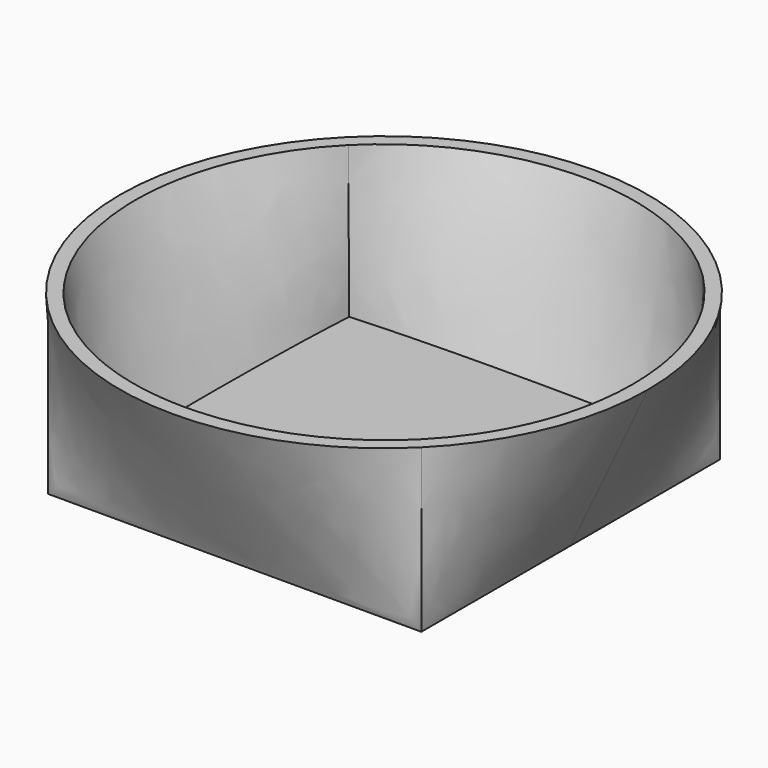
from build123d import *

# Parameters (mm, degrees)
F0_R = 48.75
F2_W = 68.9429111657
F2_H = 68.9429111657
F4_T = 2.5


# Not quite as in the source:
# - a shell that OpenCascade refuses in one call is made with other operations: the cavity is built on its own and cut out


with BuildPart() as f3:
    # F0 (on Top) → F3 section 0
    with BuildSketch(Plane.XY):
        Circle(F0_R)
    # F2 (on offset) → F3 section 1
    with BuildSketch(Plane.XY.offset(-30)):
        Rectangle(F2_W, F2_H)
    loft()

    # F4: shell of thickness 2.5, made by hand


with BuildPart() as f4_core1:
    # F4_t2: copy of F3
    add(f3.part)

    # the walls: a layer under each face that stays
    f4_faces = [f4_core1.faces().sort_by_distance(p)[0] for p in [
        (39.7552913915, 17.9457725576, -15),
        (0, 41.6107277896, -15),
        (-41.6107277896, 0, -15),
        (0, -41.6107277896, -15),
        (39.7552913915, -17.9457725576, -15),
        (0, 0, -30),
    ]]
    thicken(f4_faces, amount=-F4_T, mode=Mode.SUBTRACT)


with BuildPart() as f3_1:
    add(f3.part)

    # what is left inside the walls is the cavity
    f4_cavity = [f4_core1.part.solids().sort_by_distance(p)[0] for p in [
        (0, -15.327093, -0.025),
    ]]
    add(f4_cavity, mode=Mode.SUBTRACT)


solid = f3_1.part
